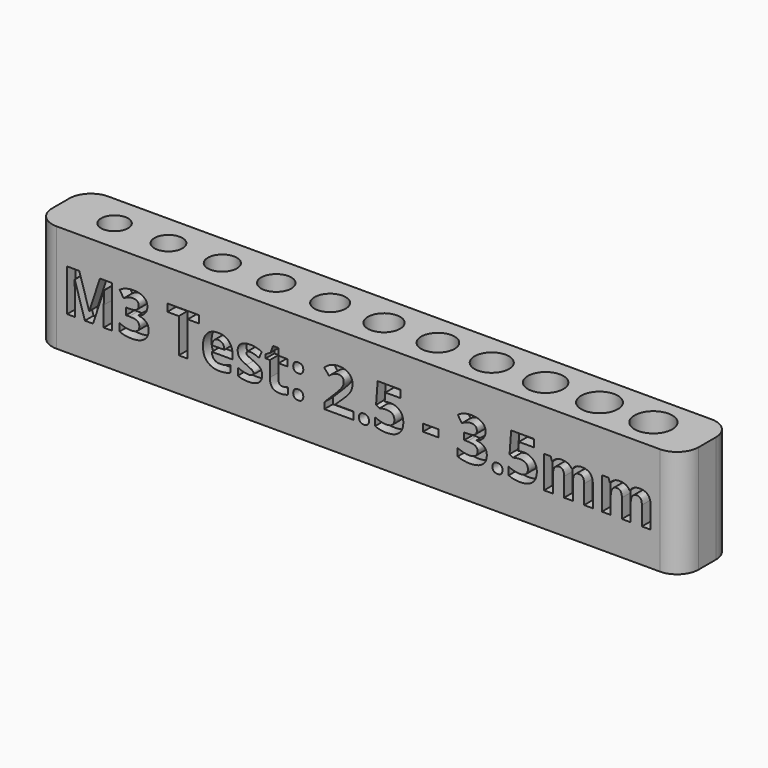
from build123d import *

# Parameters (mm, degrees)
F0_W         = 60
F0_H         = 6
F0_R         = 1.25
F0_R_2       = 1.3
F0_R_3       = 1.35
F0_R_4       = 1.4
F0_R_5       = 1.45
F0_R_6       = 1.5
F0_R_7       = 1.55
F0_R_8       = 1.6
F0_R_9       = 1.65
F0_R_10      = 1.7
F0_R_11      = 1.75
F1_DEPTH     = 10
F2_R         = 2
F3_TEXT_SIZE = 5.4627847787
F4_DEPTH     = 1


# Not quite as in the source:
# - Text() gives the source's letters only with a copy of the font that has no kerning and outlines rounded to 1/6400 em; it was checked with that copy


with BuildPart() as f1:
    # F0 (on Top) → F1 (new body)
    with BuildSketch(Plane.XY):
        Rectangle(F0_W, F0_H)
        with Locations((-25, 0)):
            Circle(F0_R, mode=Mode.SUBTRACT)
        with Locations((-20, 0)):
            Circle(F0_R_2, mode=Mode.SUBTRACT)
        with Locations((-15, 0)):
            Circle(F0_R_3, mode=Mode.SUBTRACT)
        with Locations((-10, 0)):
            Circle(F0_R_4, mode=Mode.SUBTRACT)
        with Locations((-5, 0)):
            Circle(F0_R_5, mode=Mode.SUBTRACT)
        Circle(F0_R_6, mode=Mode.SUBTRACT)
        with Locations((5, 0)):
            Circle(F0_R_7, mode=Mode.SUBTRACT)
        with Locations((10, 0)):
            Circle(F0_R_8, mode=Mode.SUBTRACT)
        with Locations((15, 0)):
            Circle(F0_R_9, mode=Mode.SUBTRACT)
        with Locations((20, 0)):
            Circle(F0_R_10, mode=Mode.SUBTRACT)
        with Locations((25, 0)):
            Circle(F0_R_11, mode=Mode.SUBTRACT)
    extrude(amount=F1_DEPTH)

    # F2
    f2_edges = [f1.edges().sort_by_distance(p)[0] for p in [
        (-30, -3, 5),
        (30, -3, 5),
        (30, 3, 5),
        (-30, 3, 5),
    ]]
    fillet(f2_edges, radius=F2_R)

    # F3 (on face) → F4 (cut)
    with BuildSketch(Plane.XZ.offset(3)):
        with Locations((-27.5, 3.1453929413)):
            Text('M3 Test: 2.5 - 3.5mm', F3_TEXT_SIZE, font='Open Sans', font_style=FontStyle.BOLD, text_align=(TextAlign.LEFT, TextAlign.BOTTOM))
    extrude(amount=-F4_DEPTH, mode=Mode.SUBTRACT)


solid = f1.part
